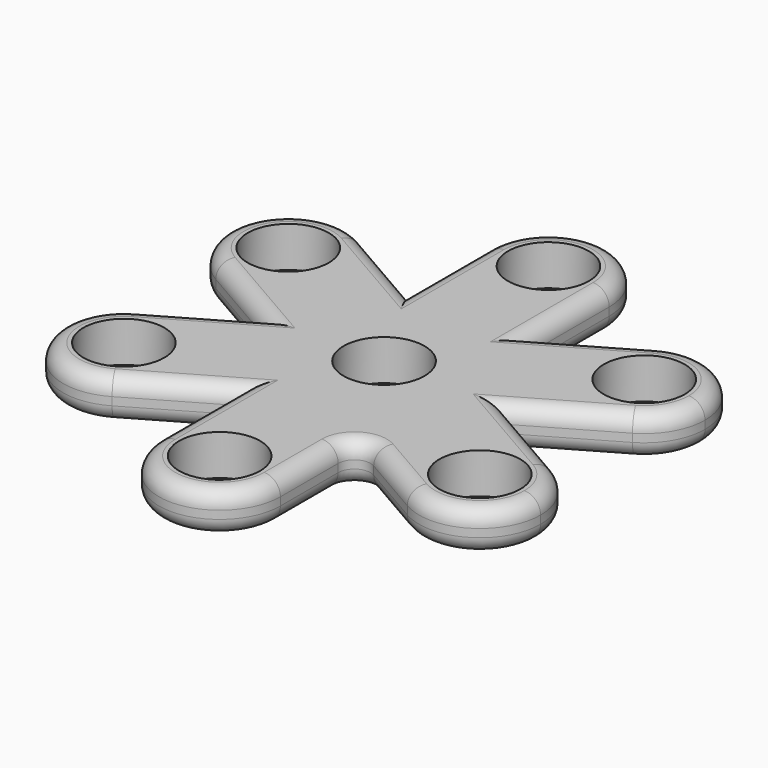
from build123d import *

# Parameters (mm, degrees)
F0_R     = 12.7
F1_DEPTH = 12.7
F2_R     = 5.08


with BuildPart() as f1:
    # F0 (on Top) → F1 (new body)
    with BuildSketch(Plane.XY):
        with BuildLine():
            ThreePointArc((-36.7565712502, 32.2199389338), (-39.3087873081, 41.7449389338), (-46.2815712502, 48.7177228759))
            ThreePointArc((-46.2815712502, 48.7177228759), (-72.3043551923, 41.7449389338), (-65.3315712502, 15.7221549918))
            ThreePointArc((-65.3315712502, 15.7221549918), (-46.2815712502, 15.7221549918), (-36.7565712502, 32.2199389338))
        make_face()
        with Locations((-55.8065712502, 32.2199389338)):
            Circle(F0_R, mode=Mode.SUBTRACT)
        with BuildLine():
            Line((-38.1, 0), (-19.05, 10.9985226281))
            Line((-19.05, 10.9985226281), (-19.05, 32.9955678842))
            Line((-19.05, 32.9955678842), (-46.2815712502, 48.7177228759))
            ThreePointArc((-46.2815712502, 48.7177228759), (-39.3087873081, 41.7449389338), (-36.7565712502, 32.2199389338))
            ThreePointArc((-36.7565712502, 32.2199389338), (-46.2815712502, 15.7221549918), (-65.3315712502, 15.7221549918))
            Line((-65.3315712502, 15.7221549918), (-38.1, 0))
        make_face()
        Polygon((-19.05, 10.9985226281), (-9.525, 16.4977839421), (0, 21.9970452561), (-19.05, 32.9955678842), align=None)
        with BuildLine():
            Line((-19.05, 32.9955678842), (0, 21.9970452561))
            Line((0, 21.9970452561), (19.05, 32.9955678842))
            Line((19.05, 32.9955678842), (19.05, 64.4398778677))
            ThreePointArc((19.05, 64.4398778677), (0, 45.3898778677), (-19.05, 64.4398778677))
            Line((-19.05, 64.4398778677), (-19.05, 32.9955678842))
        make_face()
        with BuildLine():
            ThreePointArc((-19.05, 64.4398778677), (0, 45.3898778677), (19.05, 64.4398778677))
            ThreePointArc((19.05, 64.4398778677), (0, 83.4898778677), (-19.05, 64.4398778677))
        make_face()
        with Locations((0, 64.4398778677)):
            Circle(F0_R, mode=Mode.SUBTRACT)
        with BuildLine():
            Line((19.05, 32.9955678842), (19.05, 10.9985226281))
            Line((19.05, 10.9985226281), (38.1, 0))
            Line((38.1, 0), (65.3315712502, 15.7221549918))
            ThreePointArc((65.3315712502, 15.7221549918), (39.3087873081, 22.6949389338), (46.2815712502, 48.7177228759))
            Line((46.2815712502, 48.7177228759), (19.05, 32.9955678842))
        make_face()
        with BuildLine():
            ThreePointArc((74.8565712502, 32.2199389338), (65.3315712502, 48.7177228759), (46.2815712502, 48.7177228759))
            ThreePointArc((46.2815712502, 48.7177228759), (39.3087873081, 22.6949389338), (65.3315712502, 15.7221549918))
            ThreePointArc((65.3315712502, 15.7221549918), (72.3043551923, 22.6949389338), (74.8565712502, 32.2199389338))
        make_face()
        with Locations((55.8065712502, 32.2199389338)):
            Circle(F0_R, mode=Mode.SUBTRACT)
        Polygon((0, 21.9970452561), (9.525, 16.4977839421), (19.05, 10.9985226281), (19.05, 32.9955678842), align=None)
        with BuildLine():
            ThreePointArc((9.525, 16.4977839421), (16.4977839421, 9.525), (19.05, 0))
            Line((19.05, 0), (19.05, 10.9985226281))
            Line((19.05, 10.9985226281), (9.525, 16.4977839421))
        make_face()
        with BuildLine():
            ThreePointArc((-9.525, 16.4977839421), (0, 19.05), (9.525, 16.4977839421))
            Line((9.525, 16.4977839421), (0, 21.9970452561))
            Line((0, 21.9970452561), (-9.525, 16.4977839421))
        make_face()
        with BuildLine():
            ThreePointArc((-19.05, 0), (-16.4977839421, 9.525), (-9.525, 16.4977839421))
            Line((-9.525, 16.4977839421), (-19.05, 10.9985226281))
            Line((-19.05, 10.9985226281), (-19.05, 0))
        make_face()
        with BuildLine():
            ThreePointArc((9.525, -16.4977839421), (16.4977839421, -9.525), (19.05, 0))
            ThreePointArc((19.05, 0), (16.4977839421, 9.525), (9.525, 16.4977839421))
            ThreePointArc((9.525, 16.4977839421), (0, 19.05), (-9.525, 16.4977839421))
            ThreePointArc((-9.525, 16.4977839421), (-16.4977839421, 9.525), (-19.05, 0))
            ThreePointArc((-19.05, 0), (-16.4977839421, -9.525), (-9.525, -16.4977839421))
            ThreePointArc((-9.525, -16.4977839421), (0, -19.05), (9.525, -16.4977839421))
        make_face()
        Circle(F0_R, mode=Mode.SUBTRACT)
        with BuildLine():
            Line((-19.05, -10.9985226281), (-9.525, -16.4977839421))
            ThreePointArc((-9.525, -16.4977839421), (-16.4977839421, -9.525), (-19.05, 0))
            Line((-19.05, 0), (-19.05, -10.9985226281))
        make_face()
        Polygon((-19.05, -10.9985226281), (-19.05, 0), (-19.05, 10.9985226281), (-38.1, 0), align=None)
        with BuildLine():
            Line((-19.05, -32.9955678842), (-19.05, -10.9985226281))
            Line((-19.05, -10.9985226281), (-38.1, 0))
            Line((-38.1, 0), (-65.3315712502, -15.7221549918))
            ThreePointArc((-65.3315712502, -15.7221549918), (-46.2815712502, -15.7221549918), (-36.7565712502, -32.2199389338))
            ThreePointArc((-36.7565712502, -32.2199389338), (-39.3087873081, -41.7449389338), (-46.2815712502, -48.7177228759))
            Line((-46.2815712502, -48.7177228759), (-19.05, -32.9955678842))
        make_face()
        Polygon((0, -21.9970452561), (-9.525, -16.4977839421), (-19.05, -10.9985226281), (-19.05, -32.9955678842), align=None)
        with BuildLine():
            Line((19.05, -32.9955678842), (0, -21.9970452561))
            Line((0, -21.9970452561), (-19.05, -32.9955678842))
            Line((-19.05, -32.9955678842), (-19.05, -64.4398778677))
            ThreePointArc((-19.05, -64.4398778677), (0, -45.3898778677), (19.05, -64.4398778677))
            Line((19.05, -64.4398778677), (19.05, -32.9955678842))
        make_face()
        Polygon((19.05, -10.9985226281), (9.525, -16.4977839421), (0, -21.9970452561), (19.05, -32.9955678842), align=None)
        with BuildLine():
            Line((38.1, 0), (19.05, -10.9985226281))
            Line((19.05, -10.9985226281), (19.05, -32.9955678842))
            Line((19.05, -32.9955678842), (46.2815712502, -48.7177228759))
            ThreePointArc((46.2815712502, -48.7177228759), (39.3087873081, -22.6949389338), (65.3315712502, -15.7221549918))
            Line((65.3315712502, -15.7221549918), (38.1, 0))
        make_face()
        Polygon((19.05, 10.9985226281), (19.05, 0), (19.05, -10.9985226281), (38.1, 0), align=None)
        with BuildLine():
            Line((19.05, -10.9985226281), (19.05, 0))
            ThreePointArc((19.05, 0), (16.4977839421, -9.525), (9.525, -16.4977839421))
            Line((9.525, -16.4977839421), (19.05, -10.9985226281))
        make_face()
        with BuildLine():
            Line((0, -21.9970452561), (9.525, -16.4977839421))
            ThreePointArc((9.525, -16.4977839421), (0, -19.05), (-9.525, -16.4977839421))
            Line((-9.525, -16.4977839421), (0, -21.9970452561))
        make_face()
        with BuildLine():
            ThreePointArc((-65.3315712502, -15.7221549918), (-72.3043551923, -41.7449389338), (-46.2815712502, -48.7177228759))
            ThreePointArc((-46.2815712502, -48.7177228759), (-39.3087873081, -41.7449389338), (-36.7565712502, -32.2199389338))
            ThreePointArc((-36.7565712502, -32.2199389338), (-46.2815712502, -15.7221549918), (-65.3315712502, -15.7221549918))
        make_face()
        with Locations((-55.8065712502, -32.2199389338)):
            Circle(F0_R, mode=Mode.SUBTRACT)
        with BuildLine():
            ThreePointArc((-19.05, -64.4398778677), (0, -83.4898778677), (19.05, -64.4398778677))
            ThreePointArc((19.05, -64.4398778677), (0, -45.3898778677), (-19.05, -64.4398778677))
        make_face()
        with Locations((0, -64.4398778677)):
            Circle(F0_R, mode=Mode.SUBTRACT)
        with BuildLine():
            ThreePointArc((74.8565712502, -32.2199389338), (72.3043551923, -22.6949389338), (65.3315712502, -15.7221549918))
            ThreePointArc((65.3315712502, -15.7221549918), (39.3087873081, -22.6949389338), (46.2815712502, -48.7177228759))
            ThreePointArc((46.2815712502, -48.7177228759), (65.3315712502, -48.7177228759), (74.8565712502, -32.2199389338))
        make_face()
        with Locations((55.8065712502, -32.2199389338)):
            Circle(F0_R, mode=Mode.SUBTRACT)
    extrude(amount=F1_DEPTH)

    # F2
    f2_edges = [f1.edges().sort_by_distance(p)[0] for p in [
        (51.715786, 7.861077, 12.7),
        (19.05, 48.717723, 12.7),
        (-32.665786, 40.856645, 12.7),
        (-51.715786, -7.861077, 12.7),
        (-19.05, -48.717723, 12.7),
        (32.665786, -40.856645, 12.7),
        (19.05, -32.995568, 6.35),
        (46.281571, -48.717723, 6.35),
        (32.665786, -40.856645, 0),
        (-51.715786, -7.861077, 0),
        (32.665786, 40.856645, 0),
        (-51.715786, 7.861077, 0),
        (-19.05, 48.717723, 0),
        (-72.304355, 41.744939, 0),
        (-72.304355, 41.744939, 12.7),
        (-51.715786, 7.861077, 12.7),
        (-72.304355, -41.744939, 0),
        (-72.304355, -41.744939, 12.7),
        (-32.665786, -40.856645, 0),
        (-32.665786, -40.856645, 12.7),
        (-19.05, -48.717723, 0),
        (0, -83.489878, 0),
        (0, -83.489878, 12.7),
        (72.304355, -41.744939, 0),
        (72.304355, -41.744939, 12.7),
        (51.715786, -7.861077, 0),
        (51.715786, -7.861077, 12.7),
        (51.715786, 7.861077, 0),
        (72.304355, 41.744939, 0),
        (72.304355, 41.744939, 12.7),
        (32.665786, 40.856645, 12.7),
        (19.05, 48.717723, 0),
        (0, 83.489878, 0),
        (0, 83.489878, 12.7),
        (-19.05, 48.717723, 12.7),
        (-32.665786, 40.856645, 0),
    ]]
    fillet(f2_edges, radius=F2_R)


solid = f1.part
